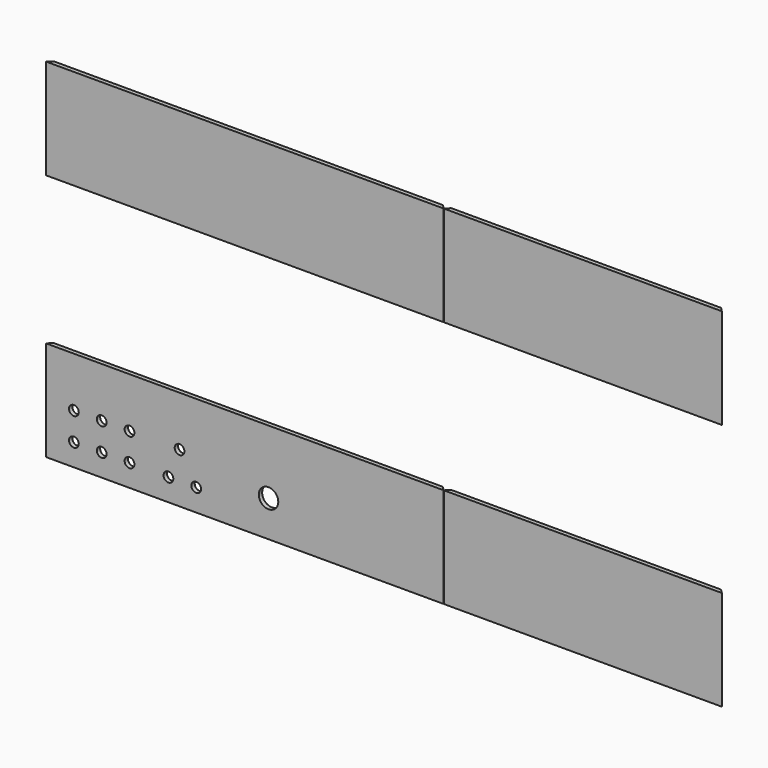
from build123d import *

# Parameters (mm, degrees)
F0_W      = 454.025
F0_H      = 114.3
F0_R      = 5.5626
F0_R_2    = 11.1125
F1_DEPTH  = 4.7752
F0_W_2    = 317.5
F2_SIZE   = 4.77519
F2_2_SIZE = 4.77519
F2_3_SIZE = 4.77519
F2_4_SIZE = 4.77519


# Not quite as in the source:
# - a fillet or chamfer is up to 0.001 mm smaller than in the source, because OpenCascade refuses the exact size
# - a feature names something its author has since deleted; it is built from what else it names


with BuildPart() as f1:
    # F0 (on Front) → F1 (new body)
    with BuildSketch(Plane.XZ):
        with Locations((37.6425363503, 2.1368730813)):
            Rectangle(F0_W, F0_H)
        with Locations((-157.6199636497, -29.6131269187)):
            Circle(F0_R, mode=Mode.SUBTRACT)
        with Locations((-125.8699636497, -29.6131269187)):
            Circle(F0_R, mode=Mode.SUBTRACT)
        with Locations((-94.1199636497, -29.6131269187)):
            Circle(F0_R, mode=Mode.SUBTRACT)
        with Locations((-49.6699636497, -29.6131269187)):
            Circle(F0_R, mode=Mode.SUBTRACT)
        with Locations((-17.9199636497, -29.6131269187)):
            Circle(F0_R, mode=Mode.SUBTRACT)
        with Locations((-157.6199636497, 2.1368730813)):
            Circle(F0_R, mode=Mode.SUBTRACT)
        with Locations((-125.8699636497, 2.1368730813)):
            Circle(F0_R, mode=Mode.SUBTRACT)
        with Locations((-94.1199636497, 2.1368730813)):
            Circle(F0_R, mode=Mode.SUBTRACT)
        with Locations((-36.9699636497, 2.1368730813)):
            Circle(F0_R, mode=Mode.SUBTRACT)
        with Locations((64.6300363503, -13.7381269187)):
            Circle(F0_R_2, mode=Mode.SUBTRACT)
    extrude(amount=F1_DEPTH)

    # F2#2 (size 4.7752 in the source; OpenCascade refuses exactly that, so slightly less here)
    f2_2_edges = [f1.edges().sort_by_distance(p)[0] for p in [
        (264.655036, 0, 2.136873),
        (-189.369964, 0, 2.136873),
    ]]
    chamfer(f2_2_edges, length=F2_2_SIZE)


with BuildPart() as f1b:
    # F0 (on Front) → F1, piece 2 (new body)
    with BuildSketch(Plane.XZ):
        with Locations((37.6425363503, 285.3470083714)):
            Rectangle(F0_W, F0_H)
    extrude(amount=F1_DEPTH)

    # F2 (size 4.7752 in the source; OpenCascade refuses exactly that, so slightly less here)
    f2_edges = [f1b.edges().sort_by_distance(p)[0] for p in [
        (264.655036, 0, 285.347008),
        (-189.369964, 0, 285.347008),
    ]]
    chamfer(f2_edges, length=F2_SIZE)


with BuildPart() as f1c:
    # F0 (on Front) → F1, piece 3 (new body)
    with BuildSketch(Plane.XZ):
        with Locations((423.5320413113, 2.1368730813)):
            Rectangle(F0_W_2, F0_H)
    extrude(amount=F1_DEPTH)

    # F2#3 (size 4.7752 in the source; OpenCascade refuses exactly that, so slightly less here)
    f2_3_edges = [f1c.edges().sort_by_distance(p)[0] for p in [
        (582.282041, 0, 2.136873),
        (264.782041, 0, 2.136873),
    ]]
    chamfer(f2_3_edges, length=F2_3_SIZE)


with BuildPart() as f1d:
    # F0 (on Front) → F1, piece 4 (new body)
    with BuildSketch(Plane.XZ):
        with Locations((423.4609160386, 285.3470083714)):
            Rectangle(F0_W_2, F0_H)
    extrude(amount=F1_DEPTH)

    # F2#4 (size 4.7752 in the source; OpenCascade refuses exactly that, so slightly less here)
    f2_4_edges = [f1d.edges().sort_by_distance(p)[0] for p in [
        (264.710916, 0, 285.347008),
        (582.210916, 0, 285.347008),
    ]]
    chamfer(f2_4_edges, length=F2_4_SIZE)


solid = Compound([f1.part, f1b.part, f1c.part, f1d.part])
